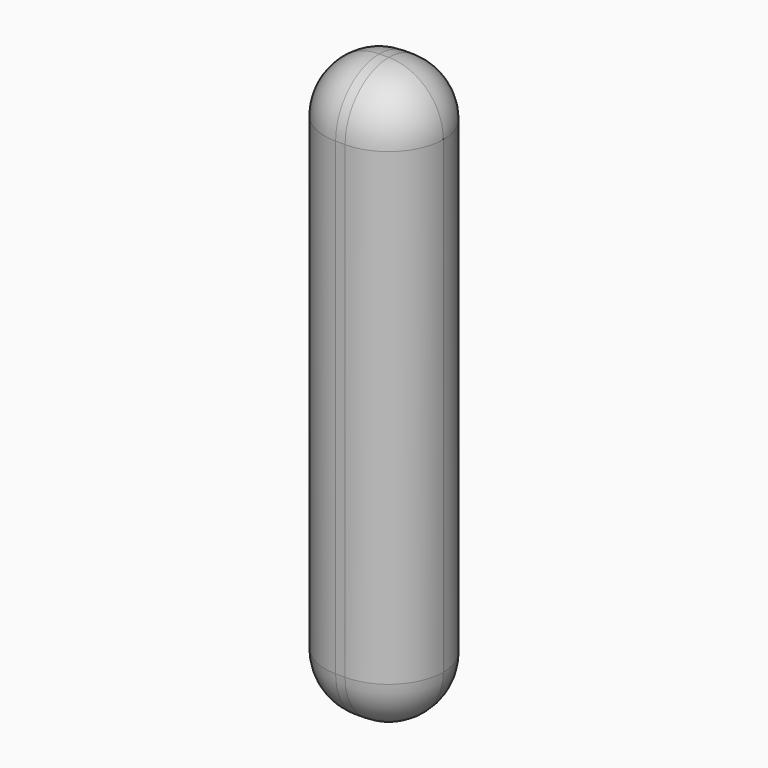
from build123d import *

# Parameters (mm, degrees)
F0_W        = 2.7607865632
F0_H        = 13.4613066912
F1_DEPTH    = 2.54
F2_R        = 1.26999
F3_T1_DEPTH = 13.4613066912
F3_T4_ANGLE = 90
F3_T6_ANGLE = 90


# Not quite as in the source:
# - a fillet or chamfer that OpenCascade refuses, or shapes differently, is made with other operations: its cross-section is extruded or revolved along the edge and cut away or added
# - a fillet or chamfer is up to 0.001 mm smaller than in the source, because OpenCascade refuses the exact size


with BuildPart() as f1:
    # F0 (on Front) → F1 (new body)
    with BuildSketch(Plane.XZ):
        with Locations((-55.148826912, 39.8645661771)):
            Rectangle(F0_W, F0_H)
    extrude(amount=F1_DEPTH)

    # F2 (radius 1.27 in the source; OpenCascade refuses exactly that, so slightly less here)
    f2_edges = [f1.edges().sort_by_distance(p)[0] for p in [
        (-55.148827, -2.54, 46.59522),
        (-53.768434, -2.54, 39.864566),
        (-56.52922, -2.54, 39.864566),
        (-55.148827, -2.54, 33.133913),
        (-55.148827, 0, 46.59522),
        (-53.768434, -1.27, 46.59522),
        (-53.768434, -1.27, 33.133913),
        (-53.768434, 0, 39.864566),
        (-55.148827, 0, 33.133913),
        (-56.52922, -1.27, 46.59522),
        (-56.52922, -1.27, 33.133913),
    ]]
    fillet(f2_edges, radius=F2_R)

    # F3: fillet of radius 1.27 on 1 edges, made by hand

    # F3_s2 → F3_t1 (cut)
    with BuildSketch(Plane.XY.offset(33.1339128315)):
        with BuildLine():
            ThreePointArc((-56.5292201936, -1.27), (-56.1572458057, -0.3719743879), (-55.2592201936, 0))
            Line((-55.2592201936, 0), (-56.5292201936, 0))
            Line((-56.5292201936, 0), (-56.5292201936, -1.27))
        make_face()
    extrude(amount=F3_T1_DEPTH, mode=Mode.SUBTRACT)

    # F3_s3 → F3_t4 (revolve, cut)
    with BuildSketch(Plane.YZ.offset(-55.2592201936)):
        with BuildLine():
            ThreePointArc((-1.26999, 46.5952195227), (-0.371971459, 46.2232480638), (0, 45.3252295227))
            Line((0, 45.3252295227), (0, 46.5952195227))
            Line((0, 46.5952195227), (-1.26999, 46.5952195227))
        make_face()
    revolve(axis=Axis((-55.2592201936, -1.27, 46.5952195227), (0, 0, 1)), revolution_arc=F3_T4_ANGLE, mode=Mode.SUBTRACT)

    # F3_s5 → F3_t6 (revolve, cut)
    with BuildSketch(Plane.XZ.offset(1.27)):
        with BuildLine():
            ThreePointArc((-55.2592301936, 33.1339128315), (-56.1572487347, 33.5058842905), (-56.5292201936, 34.4039028315))
            Line((-56.5292201936, 34.4039028315), (-56.5292201936, 33.1339128315))
            Line((-56.5292201936, 33.1339128315), (-55.2592301936, 33.1339128315))
        make_face()
    revolve(axis=Axis((-55.2592201936, -1.27, 33.1339128315), (0, 0, -1)), revolution_arc=F3_T6_ANGLE, mode=Mode.SUBTRACT)


solid = f1.part
